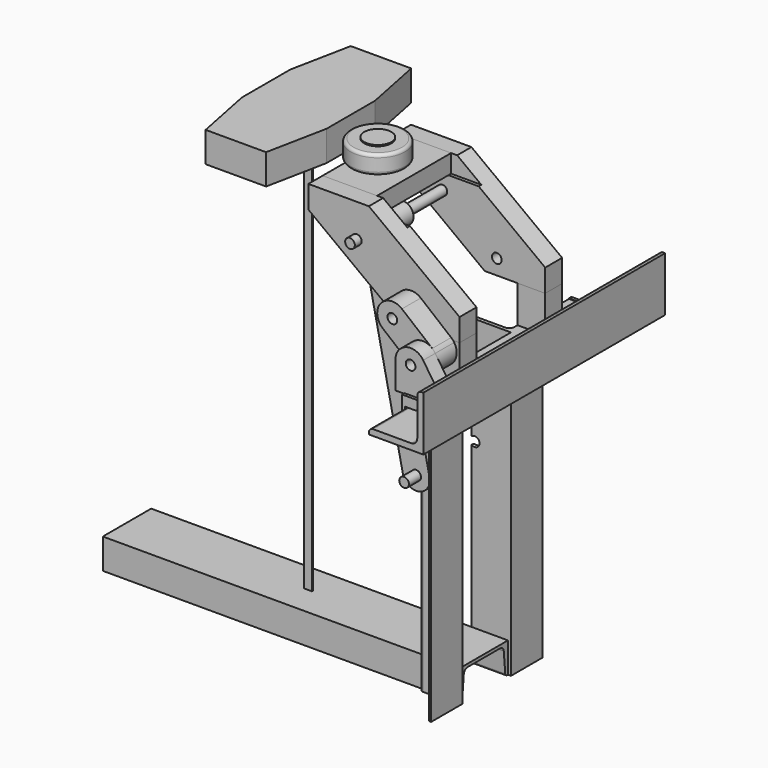
from build123d import *

# Parameters (mm, degrees)
F1_DEPTH  = 250
F2_DEPTH  = 175
F3_START  = 145
F0_R      = 8
F3_DEPTH  = 25
F4_R      = 8
F5_DEPTH  = 39
F6_R      = 8
F7_DEPTH  = 35
F8_W      = 5.5
F8_H      = 30
F9_DEPTH  = 305.2282578985
F11_DEPTH = 90
F12_R     = 17.5
F13_DEPTH = 236.259
F14_R     = 17.5
F15_DEPTH = 40
F14_R_2   = 22.5
F16_DEPTH = 35
F17_START = 2
F17_DEPTH = 31
F18_R     = 5
F19_R     = 8
F20_DEPTH = 15
F21_R     = 8
F22_DEPTH = 120
F23_START = 10.5
F21_R_2   = 17.5
F23_DEPTH = 60.5
F24_R     = 8
F25_DEPTH = 5.5
F24_W     = 90
F24_H     = 30
F26_DEPTH = 29.5
F28_DEPTH = 1
F30_DEPTH = 500
F32_DEPTH = 306.001
F34_START = -5
F34_DEPTH = 590
F35_W     = 13.3450913429
F35_H     = 664
F36_DEPTH = 1
F37_DEPTH = 150
F39_DEPTH = 50
F40_W     = 45.7727421015
F40_H     = 35
F41_DEPTH = 61.258
F42_DEPTH = 25


with BuildPart() as f1:
    # F0 (on Front) → F1 (new body, symmetric)
    with BuildSketch(Plane.XZ):
        with BuildLine():
            Line((-90, 0), (0, 0))
            Line((0, 0), (0, 90))
            Line((0, 90), (-3, 90))
            ThreePointArc((-3, 90), (-7.9497474683, 87.9497474683), (-10, 83))
            Line((-10, 83), (-10, 20))
            ThreePointArc((-10, 20), (-12.9289321881, 12.9289321881), (-20, 10))
            Line((-20, 10), (-30, 10))
            Line((-30, 10), (-83, 10))
            ThreePointArc((-83, 10), (-87.9497474683, 7.9497474683), (-90, 3))
            Line((-90, 3), (-90, 0))
        make_face()
    extrude(amount=F1_DEPTH, both=True)


with BuildPart() as f2:
    # F0 (on Front) → F2 (new body, symmetric)
    with BuildSketch(Plane.XZ):
        Polygon((-95, 0), (-90, 0), (-90, 3), (-90, 10), (-83, 10), (-30, 10), (-30, 25), (-35, 25), (-95, 25), align=None)
    extrude(amount=F2_DEPTH, both=True)

    # F27 (on face) → F28 (join)
    with BuildSketch(Plane.XY.offset(25)):
        Polygon((-35, -145), (-35, -170), (-95, -170), (-95, -175), (-30, -175), (-30, -145), align=None)
        Polygon((-95, 175), (-95, 170), (-35, 170), (-35, 145), (-30, 145), (-30, 175), align=None)
    extrude(amount=F28_DEPTH)

    # F29 (on face) → F30 (join)
    with BuildSketch(Plane.XY.offset(25)):
        with BuildLine():
            Line((-160, 50), (-95, 50))
            Line((-95, 50), (-95, 115))
            Line((-95, 115), (-97, 115))
            ThreePointArc((-97, 115), (-99.8284271247, 113.8284271247), (-101, 111))
            Line((-101, 111), (-101, 64))
            ThreePointArc((-101, 64), (-103.3431457505, 58.3431457505), (-109, 56))
            Line((-109, 56), (-156, 56))
            ThreePointArc((-156, 56), (-158.8284271247, 54.8284271247), (-160, 52))
            Line((-160, 52), (-160, 50))
        make_face()
        with BuildLine():
            Line((-95, -115), (-95, -50))
            Line((-95, -50), (-160, -50))
            Line((-160, -50), (-160, -52))
            ThreePointArc((-160, -52), (-158.8284271247, -54.8284271247), (-156, -56))
            Line((-156, -56), (-109, -56))
            ThreePointArc((-109, -56), (-103.3431457505, -58.3431457505), (-101, -64))
            Line((-101, -64), (-101, -111))
            ThreePointArc((-101, -111), (-99.8284271247, -113.8284271247), (-97, -115))
            Line((-97, -115), (-95, -115))
        make_face()
    extrude(amount=-F30_DEPTH)

    # F31 (on face) → F32 (cut, through all)
    with BuildSketch(Plane.XZ.offset(56)):
        with BuildLine():
            ThreePointArc((-156, -161.3912678318), (-149.7084973779, -159.4540138986), (-147, -153.4540138986))
            ThreePointArc((-147, -153.4540138986), (-149.7084973779, -147.4540138986), (-156, -145.5167599654))
            Line((-156, -145.5167599654), (-156, -161.3912678318))
        make_face()
        with BuildLine():
            Line((-156, -161.3912678318), (-156, -145.5167599654))
            ThreePointArc((-156, -145.5167599654), (-163, -153.4540138986), (-156, -161.3912678318))
        make_face()
    extrude(amount=-F32_DEPTH, mode=Mode.SUBTRACT)

    # F33 (on face) → F34 (join)
    with BuildSketch(Plane.YZ.offset(-95).offset(F34_START)):
        with BuildLine():
            Line((-50, -425), (-50, -475))
            Line((-50, -475), (-48.3525412842, -475))
            ThreePointArc((-48.3525412842, -475), (-45.6501804538, -473.9491093472), (-44.3677624919, -471.348622971))
            Line((-44.3677624919, -471.348622971), (-41.3891349221, -437.302754058))
            ThreePointArc((-41.3891349221, -437.302754058), (-38.8242989983, -432.1017813055), (-33.4195773373, -430))
            Line((-33.4195773373, -430), (33.4195773373, -430))
            ThreePointArc((33.4195773373, -430), (38.8242989983, -432.1017813055), (41.3891349221, -437.302754058))
            Line((41.3891349221, -437.302754058), (44.3677624919, -471.348622971))
            ThreePointArc((44.3677624919, -471.348622971), (45.6501804538, -473.9491093472), (48.3525412842, -475))
            Line((48.3525412842, -475), (50, -475))
            Line((50, -475), (50, -425))
            Line((50, -425), (-50, -425))
        make_face()
    extrude(amount=-F34_DEPTH)

    # F35 (on Front) → F36 (join, symmetric)
    with BuildSketch(Plane.XZ):
        Polygon((-460, 239), (-396.6725456715, 239), (-383.3274543285, 239), (-320, 239), (-320, 289), (-460, 289), align=None)
        with Locations((-390, -93)):
            Rectangle(F35_W, F35_H)
    extrude(amount=F36_DEPTH, both=True)

    # F35 (on Front) → F37 (join, symmetric)
    with BuildSketch(Plane.XZ):
        Polygon((-460, 239), (-396.6725456715, 239), (-383.3274543285, 239), (-320, 239), (-320, 289), (-460, 289), align=None)
    extrude(amount=F37_DEPTH, both=True)

    # F38 (on face) → F39 (cut, through all)
    with BuildSketch(Plane.XY.offset(289)):
        Polygon((-320, 150), (-340, 150), (-320, 50), align=None)
        Polygon((-440, 150), (-460, 150), (-460, 50), align=None)
        Polygon((-440, -150), (-460, -50), (-460, -150), align=None)
        Polygon((-320, -150), (-320, -50), (-340, -150), align=None)
    extrude(amount=-F39_DEPTH, mode=Mode.SUBTRACT)

    # F40 (on face) → F41 (join, through all)
    with BuildSketch(Plane.XY.offset(25)):
        with Locations((-78.1136289492, 88.5)):
            Rectangle(F40_W, F40_H)
        with Locations((-78.1136289492, -88.5)):
            Rectangle(F40_W, F40_H)
    extrude(amount=F41_DEPTH)


with BuildPart() as f3:
    # F0 (on Front) → F3 (new body)
    with BuildSketch(Plane.XZ.offset(F3_START)):
        with BuildLine():
            Line((-110, 25), (-95, 25))
            Line((-95, 25), (-35, 25))
            Line((-35, 25), (-35, 40))
            Line((-35, 40), (-64.1886171844, 83.8523046927))
            ThreePointArc((-64.1886171844, 83.8523046927), (-61.0700546345, 77.2358631002), (-60, 70))
            ThreePointArc((-60, 70), (-85, 45), (-110, 70))
            Line((-110, 70), (-110, 25))
        make_face()
        with BuildLine():
            ThreePointArc((-64.1886171844, 83.8523046927), (-92.2358631002, 93.9299453655), (-110, 70))
            ThreePointArc((-110, 70), (-85, 45), (-60, 70))
            ThreePointArc((-60, 70), (-61.0700546345, 77.2358631002), (-64.1886171844, 83.8523046927))
        make_face()
        with Locations((-85, 70)):
            Circle(F0_R, mode=Mode.SUBTRACT)
    extrude(amount=F3_DEPTH)


with BuildPart() as f5:
    # F4 (on face) → F5 (new body)
    with BuildSketch(Plane(origin=(0, -145, 0), x_dir=(-1, 0, 0), z_dir=(0, 1, 0))):
        with BuildLine():
            Line((110, 58.1827114433), (151.0957194369, 91.9398238852))
            ThreePointArc((151.0957194369, 91.9398238852), (154.5454340133, 127.1264615385), (119.35879636, 130.5761761148))
            Line((119.35879636, 130.5761761148), (69.1315384615, 89.3181761148))
            ThreePointArc((69.1315384615, 89.3181761148), (95.6838303417, 92.602118689), (110, 70))
            Line((110, 70), (110, 58.1827114433))
        make_face()
        with Locations((135.2272578985, 111.258)):
            Circle(F4_R, mode=Mode.SUBTRACT)
        with BuildLine():
            Line((100.8684615385, 50.6818238852), (110, 58.1827114433))
            Line((110, 58.1827114433), (110, 70))
            ThreePointArc((110, 70), (95.6838303417, 92.602118689), (69.1315384615, 89.3181761148))
            ThreePointArc((69.1315384615, 89.3181761148), (66.4575707346, 86.7683725191), (64.1886171844, 83.8523046927))
            ThreePointArc((64.1886171844, 83.8523046927), (68.2316274809, 51.4575707346), (100.8684615385, 50.6818238852))
        make_face()
        with Locations((85, 70)):
            Circle(F4_R, mode=Mode.SUBTRACT)
    extrude(amount=F5_DEPTH)


with BuildPart() as f7:
    # F6 (on face) → F7 (new body)
    with BuildSketch(Plane(origin=(0, -106, 0), x_dir=(-1, 0, 0), z_dir=(0, 1, 0))):
        with BuildLine():
            Line((55.2272578985, 123.758), (55.2272578985, 86.258))
            Line((55.2272578985, 86.258), (66.0084904234, 86.258))
            ThreePointArc((66.0084904233, 86.258), (67.502984083, 87.8564955688), (69.1315384615, 89.3181761148))
            Line((69.1315384615, 89.3181761148), (119.35879636, 130.5761761148))
            ThreePointArc((119.35879636, 130.5761761148), (154.5454340133, 127.1264615385), (151.0957194369, 91.9398238852))
            Line((151.0957194369, 91.9398238852), (144.1786988927, 86.258))
            Line((144.1786988927, 86.258), (155.2272578985, 86.258))
            Line((155.2272578985, 86.258), (305.2272578985, 198.758))
            Line((305.2272578985, 198.758), (305.2272578985, 236.258))
            Line((305.2272578985, 236.258), (205.2272578985, 236.258))
            Line((205.2272578985, 236.258), (55.2272578985, 123.758))
        make_face()
        with Locations((225.2272578985, 181.258)):
            Circle(F6_R, mode=Mode.SUBTRACT)
        with BuildLine():
            ThreePointArc((69.1315384615, 89.3181761148), (67.502984083, 87.8564955688), (66.0084904233, 86.258))
            Line((66.0084904234, 86.258), (144.1786988927, 86.258))
            Line((144.1786988927, 86.258), (151.0957194369, 91.9398238852))
            ThreePointArc((151.0957194369, 91.9398238852), (154.5454340133, 127.1264615385), (119.35879636, 130.5761761148))
            Line((119.35879636, 130.5761761148), (69.1315384615, 89.3181761148))
        make_face()
        with Locations((135.2272578985, 111.258)):
            Circle(F6_R, mode=Mode.SUBTRACT)
    extrude(amount=F7_DEPTH)

    # F8 (on face) → F9 (cut, through all)
    with BuildSketch(Plane(origin=(-305.2272578985, 0, 0), x_dir=(0, -1, 0), z_dir=(-1, 0, 0))):
        with Locations((73.75, 221.258)):
            Rectangle(F8_W, F8_H)
    extrude(amount=-F9_DEPTH, mode=Mode.SUBTRACT)


with BuildPart() as f11:
    # F10 (on face) → F11 (new body)
    with BuildSketch(Plane(origin=(-305.2272578985, 0, 0), x_dir=(0, -1, 0), z_dir=(-1, 0, 0))):
        Polygon((76.5, 206.258), (76.5, 236.258), (-76.5, 236.258), (-76.5, 206.258), (71, 206.258), align=None)
    extrude(amount=-F11_DEPTH)

    # F12 (on face) → F13 (cut, through all)
    with BuildSketch(Plane.XY.offset(236.258)):
        with Locations((-275.2272578985, 0)):
            Circle(F12_R)
    extrude(amount=-F13_DEPTH, mode=Mode.SUBTRACT)


with BuildPart() as f15:
    # F14 (on face) → F15 (new body)
    with BuildSketch(Plane.XY.offset(236.258)):
        with Locations((-275.2272578985, 0)):
            Circle(F14_R)
    extrude(amount=-F15_DEPTH)

    # F14 (on face) → F16 (join)
    with BuildSketch(Plane.XY.offset(236.258)):
        with Locations((-275.2272578985, 0)):
            Circle(F14_R_2)
        with Locations((-275.2272578985, 0)):
            Circle(F14_R, mode=Mode.SUBTRACT)
        with Locations((-275.2272578985, 0)):
            Circle(F14_R)
    extrude(amount=F16_DEPTH)

    # F14 (on face) → F17 (join)
    with BuildSketch(Plane.XY.offset(236.258).offset(F17_START)):
        with BuildLine():
            ThreePointArc((-305.2272578985, -33.5410196625), (-256.8560848276, -41.0791918129), (-230.2272578985, 0))
            ThreePointArc((-230.2272578985, 0), (-256.8560848276, 41.0791918129), (-305.2272578985, 33.5410196625))
            Line((-305.2272578985, 33.5410196625), (-305.2272578985, -33.5410196625))
        make_face()
        with Locations((-275.2272578985, 0)):
            Circle(F14_R_2, mode=Mode.SUBTRACT)
        with BuildLine():
            Line((-305.2272578985, -33.5410196625), (-305.2272578985, 33.5410196625))
            ThreePointArc((-305.2272578985, 33.5410196625), (-320.2272578985, 0), (-305.2272578985, -33.5410196625))
        make_face()
        with Locations((-275.2272578985, 0)):
            Circle(F14_R_2)
        with Locations((-275.2272578985, 0)):
            Circle(F14_R, mode=Mode.SUBTRACT)
        with Locations((-275.2272578985, 0)):
            Circle(F14_R)
    extrude(amount=F17_DEPTH)

    # F18
    f18_edges = [f15.edges().sort_by_distance(p)[0] for p in [
        (-320.227258, 0, 269.258),
        (-320.227258, 0, 238.258),
    ]]
    fillet(f18_edges, radius=F18_R)


with BuildPart() as f20:
    # F19 (on face) → F20 (new body)
    with BuildSketch(Plane(origin=(0, -71, 0), x_dir=(-1, 0, 0), z_dir=(0, 1, 0))):
        with BuildLine():
            Line((177.0205272302, -158.074228234), (241.9281347635, 151.2836576488))
            Line((241.9281347635, 151.2836576488), (187.3617104804, 110.3588394364))
            Line((187.3617104804, 110.3588394364), (132.9794727698, -148.8337995632))
            ThreePointArc((132.9794727698, -148.8337995632), (150.3797856646, -175.4745411288), (177.0205272302, -158.074228234))
        make_face()
        with Locations((155, -153.4540138986)):
            Circle(F19_R, mode=Mode.SUBTRACT)
        with BuildLine():
            Line((241.9281347635, 151.2836576488), (247.2477851286, 176.6377856646))
            ThreePointArc((247.2477851286, 176.6377856646), (229.8474722339, 203.2785272302), (203.2067306683, 185.8782143354))
            Line((203.2067306683, 185.8782143354), (187.3617104804, 110.3588394364))
            Line((187.3617104804, 110.3588394364), (241.9281347635, 151.2836576488))
        make_face()
        with Locations((225.2272578985, 181.258)):
            Circle(F19_R, mode=Mode.SUBTRACT)
    extrude(amount=F20_DEPTH)

    # F19 (on face) → F42 (join, symmetric)
    with BuildSketch(Plane(origin=(0, -71, 0), x_dir=(-1, 0, 0), z_dir=(0, 1, 0))):
        with Locations((225.2272578985, 181.258)):
            Circle(F19_R)
        with Locations((155, -153.4540138986)):
            Circle(F19_R)
    extrude(amount=F42_DEPTH, both=True)


with BuildPart() as f22:
    # F21 (on Front) → F22 (new body, symmetric)
    with BuildSketch(Plane.XZ):
        with Locations((-225.2272578985, 181.258)):
            Circle(F21_R)
    extrude(amount=F22_DEPTH, both=True)


with BuildPart() as f23:
    # F21 (on Front) → F23 (new body)
    with BuildSketch(Plane.XZ.offset(F23_START)):
        with Locations((-225.2272578985, 181.258)):
            Circle(F21_R_2)
        with Locations((-225.2272578985, 181.258)):
            Circle(F21_R, mode=Mode.SUBTRACT)
    extrude(amount=F23_DEPTH)


with BuildPart() as f25:
    # F24 (on face) → F25 (new body)
    with BuildSketch(Plane(origin=(0, 76.5, 0), x_dir=(-1, 0, 0), z_dir=(0, 1, 0))):
        Polygon((215.2272578985, 206.258), (165.2272578985, 206.258), (55.2272578985, 123.758), (55.2272578985, 86.258), (155.2272578985, 86.258), (305.2272578985, 198.758), (305.2272578985, 206.258), align=None)
        with Locations((135.2272578985, 111.258)):
            Circle(F24_R, mode=Mode.SUBTRACT)
        with Locations((225.2272578985, 181.258)):
            Circle(F24_R, mode=Mode.SUBTRACT)
    extrude(amount=-F25_DEPTH)

    # F24 (on face) → F26 (join)
    with BuildSketch(Plane(origin=(0, 76.5, 0), x_dir=(-1, 0, 0), z_dir=(0, 1, 0))):
        Polygon((215.2272578985, 206.258), (165.2272578985, 206.258), (55.2272578985, 123.758), (55.2272578985, 86.258), (155.2272578985, 86.258), (305.2272578985, 198.758), (305.2272578985, 206.258), align=None)
        with Locations((135.2272578985, 111.258)):
            Circle(F24_R, mode=Mode.SUBTRACT)
        with Locations((225.2272578985, 181.258)):
            Circle(F24_R, mode=Mode.SUBTRACT)
        Polygon((215.2272578985, 236.258), (205.2272578985, 236.258), (165.2272578985, 206.258), (215.2272578985, 206.258), align=None)
        with Locations((260.2272578985, 221.258)):
            Rectangle(F24_W, F24_H)
    extrude(amount=F26_DEPTH)


solid = Compound([f1.part, f2.part, f3.part, f5.part, f7.part, f11.part, f15.part, f20.part, f22.part, f23.part, f25.part])
